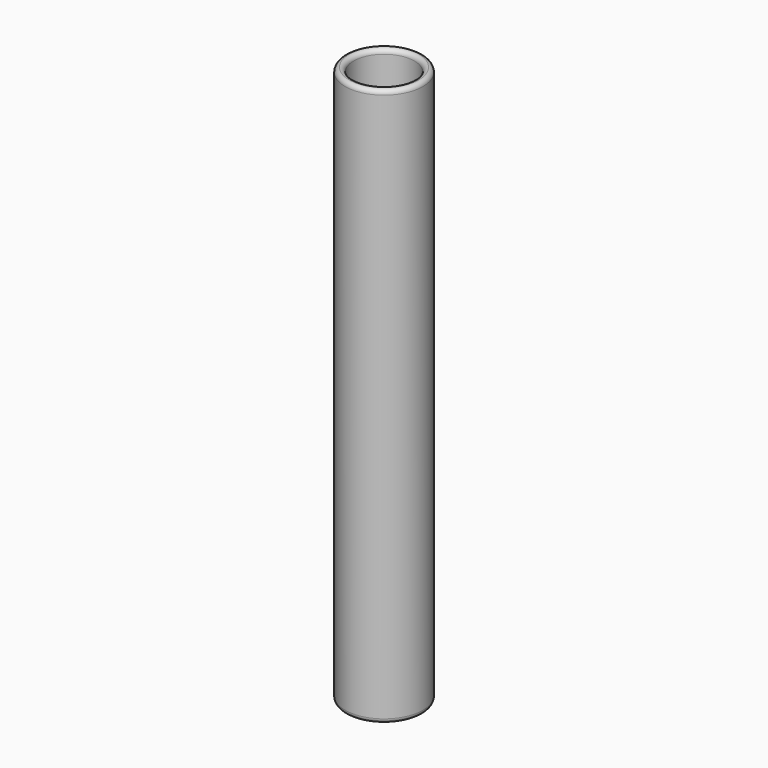
from build123d import *

# Parameters (mm, degrees)
F0_R     = 17.45
F0_R_2   = 13.6
F1_DEPTH = 250
F2_R     = 2
F4_R     = 2


# Not quite as in the source:
# - a fillet or chamfer that OpenCascade refuses, or shapes differently, is made with other operations: its cross-section is extruded or revolved along the edge and cut away or added


with BuildPart() as f1:
    # F0 (on Top) → F1 (new body)
    with BuildSketch(Plane.XY):
        Circle(F0_R)
        Circle(F0_R_2, mode=Mode.SUBTRACT)
    extrude(amount=F1_DEPTH)

    # F2
    f2_edges = [f1.edges().sort_by_distance(p)[0] for p in [
        (-13.6, 0, 250),
    ]]
    fillet(f2_edges, radius=F2_R)

    # F3: fillet of radius 2 on 1 edges, made by hand

    # F3_s1 → F3_t2 (revolve, cut)
    with BuildSketch(Plane.XZ):
        with BuildLine():
            ThreePointArc((15.6, 250), (16.9162878299, 249.3657799834), (17.45, 248.0056329325))
            Line((17.45, 248.0056329325), (17.45, 250))
            Line((17.45, 250), (15.6, 250))
        make_face()
    revolve(axis=Axis((0, 0, 250), (0, 0, 1)), mode=Mode.SUBTRACT)

    # F4
    f4_edges = [f1.edges().sort_by_distance(p)[0] for p in [
        (-13.6, 0, 0),
    ]]
    fillet(f4_edges, radius=F4_R)

    # F5: fillet of radius 2 on 1 edges, made by hand

    # F5_s1 → F5_t2 (revolve, cut)
    with BuildSketch(Plane.XZ):
        with BuildLine():
            ThreePointArc((15.6, 0), (16.9162878299, 0.6342200166), (17.45, 1.9943670675))
            Line((17.45, 1.9943670675), (17.45, 0))
            Line((17.45, 0), (15.6, 0))
        make_face()
    revolve(axis=Axis((0, 0, 0), (0, 0, 1)), mode=Mode.SUBTRACT)


solid = f1.part
